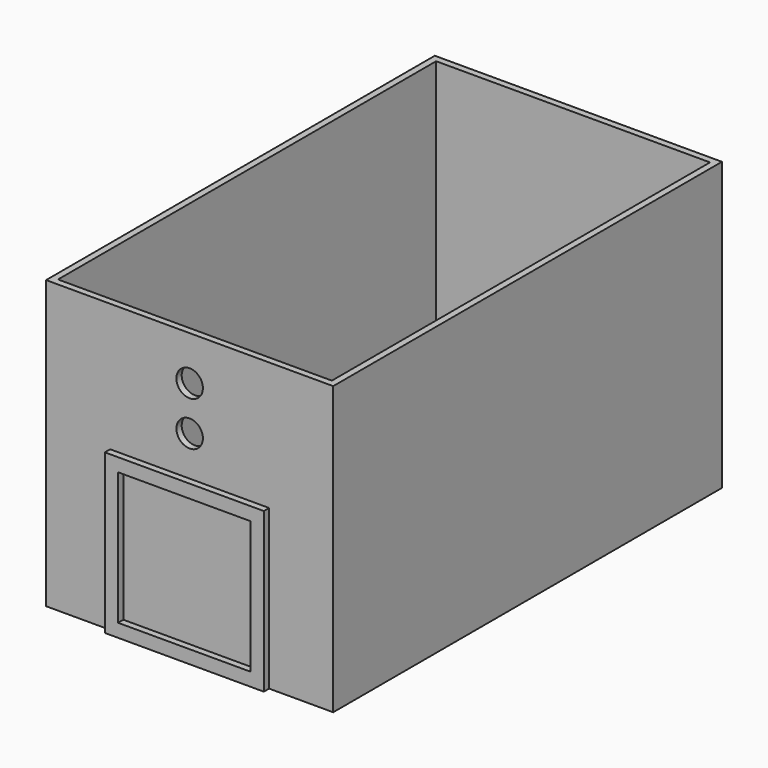
from build123d import *

# Parameters (mm, degrees)
F0_W         = 65
F0_H         = 65
F1_DEPTH     = 55
F2_W         = 36
F2_H         = 36
F2_W_2       = 30
F2_H_2       = 30
F3_DEPTH     = 1.5
F5_T         = 1.5
F5_T3_DEPTH  = 39
F5_T5_DEPTH  = 39
F5_T7_DEPTH  = 4.5
F5_T9_DEPTH  = 33
F5_T11_DEPTH = 33
F5_T13_DEPTH = 4.5
F6_R         = 3
F7_DEPTH     = 1.5


# Not quite as in the source:
# - a shell that OpenCascade refuses in one call is made with other operations: the cavity is built on its own and cut out


with BuildPart() as f1:
    # F0 (on Front) → F1 (new body)
    with BuildSketch(Plane.XZ):
        with Locations((0, 32.5)):
            Rectangle(F0_W, F0_H)
    extrude(amount=F1_DEPTH)

    # F2 (on face) → F3 (join)
    with BuildSketch(Plane.XZ.offset(55)):
        with Locations((0, 18)):
            Rectangle(F2_W, F2_H)
        with Locations((0, 18)):
            Rectangle(F2_W_2, F2_H_2, mode=Mode.SUBTRACT)
    extrude(amount=F3_DEPTH)

    # F4: F1 across plane


with BuildPart() as f1_1:
    add(f1.part)
    add(f1.part.mirror(Plane.XZ))

    # F5: shell of thickness 1.5, made by hand


with BuildPart() as f5_core1:
    # F5_t2: copy of F1
    add(f1_1.part)

    # the walls: a layer under each face that stays
    f5_faces = [f5_core1.faces().sort_by_distance(p)[0] for p in [
        (-21.6666666667, 55, 10.8333333333),
        (-18, 55.75, 18),
        (-15.4285714286, 56.5, 2.5714285714),
        (0, 55.75, 3),
        (0, 55, 18),
        (15, 55.75, 18),
        (0, 55.75, 33),
        (-15, 55.75, 18),
        (0, 55.75, 36),
        (18, 55.75, 18),
        (0, 0, 0),
        (18, -55.75, 18),
        (0, -55.75, 36),
        (-15.4285714286, -56.5, 2.5714285714),
        (0, -55.75, 3),
        (0, -55, 18),
        (15, -55.75, 18),
        (0, -55.75, 33),
        (-15, -55.75, 18),
        (-18, -55.75, 18),
        (-32.5, 0, 32.5),
        (-21.6666666667, -55, 10.8333333333),
        (32.5, 0, 32.5),
    ]]
    thicken(f5_faces, amount=-F5_T, mode=Mode.SUBTRACT)

    # F5_s4 → F5_t3 (cut)
    with BuildSketch(Plane.XY.offset(-1.5)):
        Polygon((18.015, 55.015), (18, 53.5), (16.5, 53.5), (16.5, 55), align=None)
        Polygon((-18.015, 55.015), (-18, 53.5), (-16.5, 53.5), (-16.5, 55), align=None)
        Polygon((18.015, -55.015), (16.5, -55), (16.5, -53.5), (18, -53.5), align=None)
        Polygon((-18.015, -55.015), (-16.5, -55), (-16.5, -53.5), (-18, -53.5), align=None)
    extrude(amount=F5_T3_DEPTH, mode=Mode.SUBTRACT)

    # F5_s6 → F5_t5 (cut)
    with BuildSketch(Plane.YZ.offset(-19.5)):
        Polygon((55.015, 36.015), (53.5, 36), (53.5, 34.5), (55, 34.5), align=None)
        Polygon((-55.015, 36.015), (-55, 34.5), (-53.5, 34.5), (-53.5, 36), align=None)
    extrude(amount=F5_T5_DEPTH, mode=Mode.SUBTRACT)

    # F5_s8 → F5_t7 (cut)
    with BuildSketch(Plane.XZ.offset(-58)):
        Polygon((14.985, 3.015), (15, 1.5), (16.5, 1.5), (16.5, 3), align=None)
        Polygon((-14.985, 3.015), (-15, 1.5), (-16.5, 1.5), (-16.5, 3), align=None)
        Polygon((14.985, 32.985), (16.5, 33), (16.5, 34.5), (15, 34.5), align=None)
        Polygon((-14.985, 32.985), (-15, 34.5), (-16.5, 34.5), (-16.5, 33), align=None)
    extrude(amount=F5_T7_DEPTH, mode=Mode.SUBTRACT)

    # F5_s10 → F5_t9 (cut)
    with BuildSketch(Plane.YZ.offset(-16.5)):
        Polygon((55.015, 3.015), (55, 1.5), (53.5, 1.5), (53.5, 3), align=None)
        Polygon((55.015, 32.985), (53.5, 33), (53.5, 34.5), (55, 34.5), align=None)
        Polygon((-55.015, 3.015), (-55, 1.5), (-53.5, 1.5), (-53.5, 3), align=None)
        Polygon((-55.015, 32.985), (-53.5, 33), (-53.5, 34.5), (-55, 34.5), align=None)
    extrude(amount=F5_T9_DEPTH, mode=Mode.SUBTRACT)

    # F5_s12 → F5_t11 (cut)
    with BuildSketch(Plane.XY.offset(1.5)):
        Polygon((-14.985, 55.015), (-15, 53.5), (-16.5, 53.5), (-16.5, 55), align=None)
        Polygon((14.985, 55.015), (15, 53.5), (16.5, 53.5), (16.5, 55), align=None)
        Polygon((-14.985, -55.015), (-15, -53.5), (-16.5, -53.5), (-16.5, -55), align=None)
        Polygon((14.985, -55.015), (15, -53.5), (16.5, -53.5), (16.5, -55), align=None)
    extrude(amount=F5_T11_DEPTH, mode=Mode.SUBTRACT)

    # F5_s14 → F5_t13 (cut)
    with BuildSketch(Plane.XZ.offset(53.5)):
        Polygon((14.985, 3.015), (15, 1.5), (16.5, 1.5), (16.5, 3), align=None)
        Polygon((-14.985, 3.015), (-15, 1.5), (-16.5, 1.5), (-16.5, 3), align=None)
        Polygon((14.985, 32.985), (16.5, 33), (16.5, 34.5), (15, 34.5), align=None)
        Polygon((-14.985, 32.985), (-15, 34.5), (-16.5, 34.5), (-16.5, 33), align=None)
    extrude(amount=F5_T13_DEPTH, mode=Mode.SUBTRACT)


with BuildPart() as f1_2:
    add(f1_1.part)

    # what is left inside the walls is the cavity
    f5_cavity = [f5_core1.part.solids().sort_by_distance(p)[0] for p in [
        (-30.985, -17.833333, 33.25),
    ]]
    add(f5_cavity, mode=Mode.SUBTRACT)

    # F6 (on face) → F7 (cut, through all)
    with BuildSketch(Plane.XZ.offset(55)):
        with Locations((0, 55)):
            Circle(F6_R)
        with Locations((0, 45)):
            Circle(F6_R)
    extrude(amount=-F7_DEPTH, mode=Mode.SUBTRACT)


solid = f1_2.part
